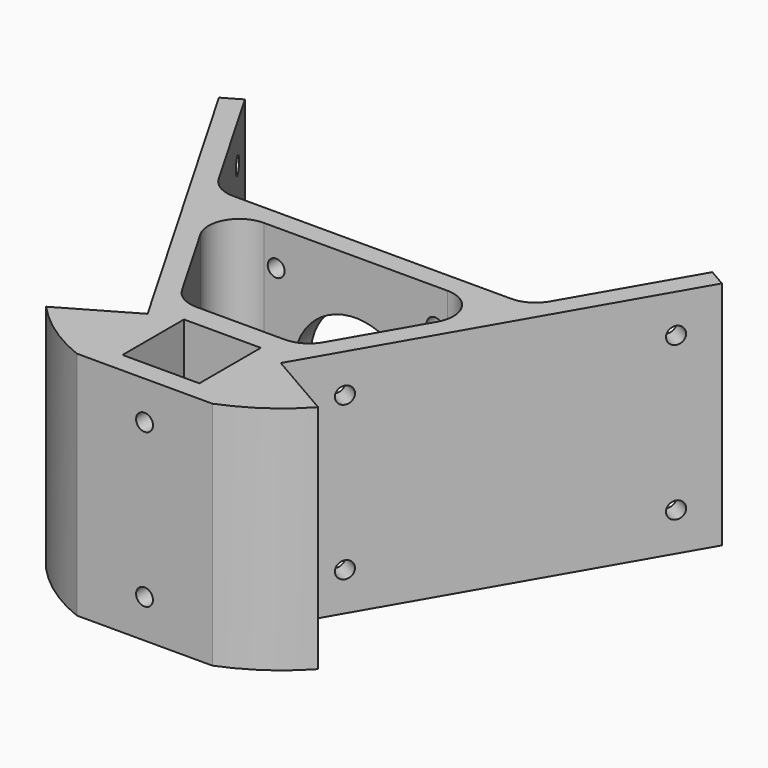
from build123d import *

# Parameters (mm, degrees)
F0_W      = 15
F0_H      = 15
F1_DEPTH  = 22.5
F2_R      = 12
F3_DEPTH  = 4
F4_D      = 3.3
F4_DEPTH  = 4
F4_TIP    = 0.9914200214
F6_D      = 3.3
F6_DEPTH  = 4
F6_TIP    = 0.9914200214
F7_R      = 6
F9_DEPTH  = 45
F11_D     = 3.3
F11_DEPTH = 4
F11_TIP   = 0.9914200214


# Not quite as in the source:
# - a pattern or mirror of a feature is missing from the dataset's text; its kind, count and spacing are read off the source's solid


with BuildPart() as f1:
    # F0 (on Top) → F1 (new body, symmetric)
    with BuildSketch(Plane.XY):
        with BuildLine():
            Line((-30.5995642671, 43.9848275573), (-45.610671266, 69.9848275573))
            Line((-45.610671266, 69.9848275573), (-49.0747728811, 67.9848275573))
            Line((-49.0747728811, 67.9848275573), (-12.9903810568, 5.4848275573))
            Line((-12.9903810568, 5.4848275573), (-26.5403215145, -2.3382342135))
            ThreePointArc((-26.5403215145, -2.3382342135), (-14.4977545891, -10.966881228), (0, -14.0151724427))
            ThreePointArc((0, -14.0151724427), (14.4977545891, -10.966881228), (26.5403215145, -2.3382342135))
            Line((26.5403215145, -2.3382342135), (12.9903810568, 5.4848275573))
            Line((12.9903810568, 5.4848275573), (49.0747728811, 67.9848275573))
            Line((49.0747728811, 67.9848275573), (45.610671266, 69.9848275573))
            Line((45.610671266, 69.9848275573), (30.5995642671, 43.9848275573))
            Line((30.5995642671, 43.9848275573), (28.2901631903, 39.9848275573))
            Line((28.2901631903, 39.9848275573), (12.0753804399, 11.9))
            Line((12.0753804399, 11.9), (0, 11.9))
            Line((0, 11.9), (-12.0753804399, 11.9))
            Line((-12.0753804399, 11.9), (-28.2901631903, 39.9848275573))
            Line((-28.2901631903, 39.9848275573), (-30.5995642671, 43.9848275573))
        make_face()
        Rectangle(F0_W, F0_H, mode=Mode.SUBTRACT)
        Polygon((0, 43.9848275573), (-30.5995642671, 43.9848275573), (-28.2901631903, 39.9848275573), (0, 39.9848275573), (28.2901631903, 39.9848275573), (30.5995642671, 43.9848275573), align=None)
    extrude(amount=F1_DEPTH, both=True)

    # F2 (on face) → F3 (cut, through all)
    with BuildSketch(Plane(origin=(0, 43.9848275573, 0), x_dir=(-1, 0, 0), z_dir=(0, 1, 0))):
        Circle(F2_R)
    extrude(amount=-F3_DEPTH, mode=Mode.SUBTRACT)

    # F4
    with Locations(Plane(origin=(0, 43.9848275573, 0), x_dir=(-1, 0, 0), z_dir=(0, 1, 0))):
        with Locations((15.5, 15.5), (15.5, -15.5), (-15.5, -15.5), (-15.5, 15.5)):
            Hole(F4_D / 2, depth=F4_DEPTH)
            with Locations((0, 0, -(F4_DEPTH + F4_TIP / 2))):  # 118° drill point
                Cone(0, F4_D / 2, F4_TIP, mode=Mode.SUBTRACT)

    # F6
    with Locations(Plane(origin=(-7.3677857926, -4.2537931107, 0), x_dir=(0.5, -0.8660254038, 0), z_dir=(-0.8660254038, -0.5, 0))):
        with Locations((-21.7451905284, -15), (-75.9139741771, -15), (-75.9139741771, 15), (-21.7451905284, 15)):
            f6 = Hole(F6_D / 2, depth=F6_DEPTH)
            with Locations((0, 0, -(F6_DEPTH + F6_TIP / 2))):  # 118° drill point
                Cone(0, F6_D / 2, F6_TIP, mode=Mode.SUBTRACT)

    # F6_copies: F6 across plane
    add(f6.mirror(Plane(origin=(0, 0, 0), x_dir=(0, 0, 1), z_dir=(1, 0, 0))), mode=Mode.SUBTRACT)

    # F7
    f7_edges = [f1.edges().sort_by_distance(p)[0] for p in [
        (-28.290163, 39.984828, 0),
        (-12.07538, 11.9, 0),
        (12.07538, 11.9, 0),
        (28.290163, 39.984828, 0),
        (-30.599564, 43.984828, 0),
        (30.599564, 43.984828, 0),
    ]]
    fillet(f7_edges, radius=F7_R)

    # F8 (on face) → F9 (cut, through all)
    with BuildSketch(Plane.XY.offset(22.5)):
        with BuildLine():
            Line((13.2199214619, -11.5), (-13.2199214619, -11.5))
            ThreePointArc((-13.2199214619, -11.5), (0, -14.0151724427), (13.2199214619, -11.5))
        make_face()
    extrude(amount=-F9_DEPTH, mode=Mode.SUBTRACT)

    # F11
    with Locations(Plane.XZ.offset(11.5)):
        with Locations((0, 15), (0, -15)):
            Hole(F11_D / 2, depth=F11_DEPTH)
            with Locations((0, 0, -(F11_DEPTH + F11_TIP / 2))):  # 118° drill point
                Cone(0, F11_D / 2, F11_TIP, mode=Mode.SUBTRACT)


solid = f1.part
